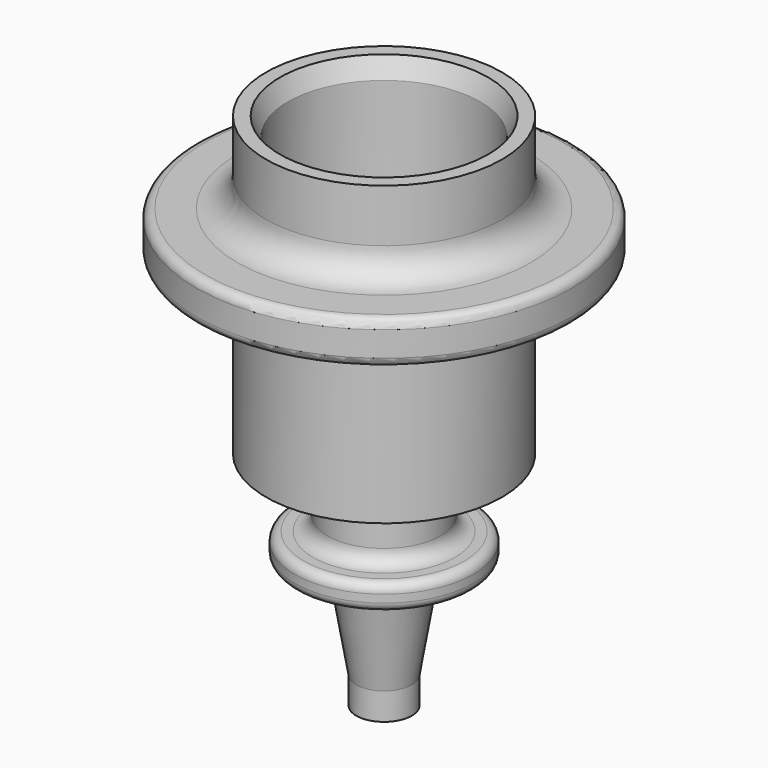
from build123d import *

# Parameters (mm, degrees)
F2_R     = 0.25
F3_R     = 0.8
F4_R     = 0.4
F5_R     = 0.125
F6_DEPTH = 2


# Not quite as in the source:
# - a feature names something its author has since deleted; it is built from what else it names


with BuildPart() as f1:
    # F0 (on Front) → F1 (revolve)
    with BuildSketch(Plane.XZ):
        Polygon((0.775, 0), (0.775, 0.76), (1.25, 3.57), (2.5, 3.57), (2.5, 4.29), (1.585, 4.29), (1.585, 5.66), (2.0212914647, 5.66), (3.3, 6.2), (3.3, 11.03), (5.255, 11.03), (5.255, 12.23), (3.3, 12.23), (3.3, 14.51), (2.9131607153, 14.51), (2.69, 13.9845872594), (2.69, 6.5387575887), (1.062589062, 5.9886043891), (0.3363867047, 1.1032430921), (0.1282693364, 1.1032430921), (0.125, 0), align=None)
    revolve(axis=Axis((0, 0, 0.6179462071), (0, 0, 1)))

    # F2
    f2_edges = [f1.edges().sort_by_distance(p)[0] for p in [
        (-5.255, 0, 12.23),
        (-5.255, 0, 11.03),
        (-2.5, 0, 4.29),
        (-2.5, 0, 3.57),
    ]]
    fillet(f2_edges, radius=F2_R)

    # F3
    f3_edges = [f1.edges().sort_by_distance(p)[0] for p in [
        (-3.3, 0, 12.23),
        (-3.3, 0, 11.03),
    ]]
    fillet(f3_edges, radius=F3_R)

    # F4
    f4_edges = [f1.edges().sort_by_distance(p)[0] for p in [
        (-1.585, 0, 4.29),
        (-1.25, 0, 3.57),
    ]]
    fillet(f4_edges, radius=F4_R)

    # F5 (on face) → F6 (cut)
    with BuildSketch(Plane(origin=(0, 0, 0), x_dir=(1, 0, 0), z_dir=(0, 0, -1))):
        with Locations((0, 0.4)):
            Circle(F5_R)
        with Locations((-0.3464101615, 0.2)):
            Circle(F5_R)
        with Locations((-0.3464101615, -0.2)):
            Circle(F5_R)
        with Locations((0, -0.4)):
            Circle(F5_R)
        with Locations((0.3464101615, -0.2)):
            Circle(F5_R)
        with Locations((0.3464101615, 0.2)):
            Circle(F5_R)
    extrude(amount=-F6_DEPTH, mode=Mode.SUBTRACT)


solid = f1.part
